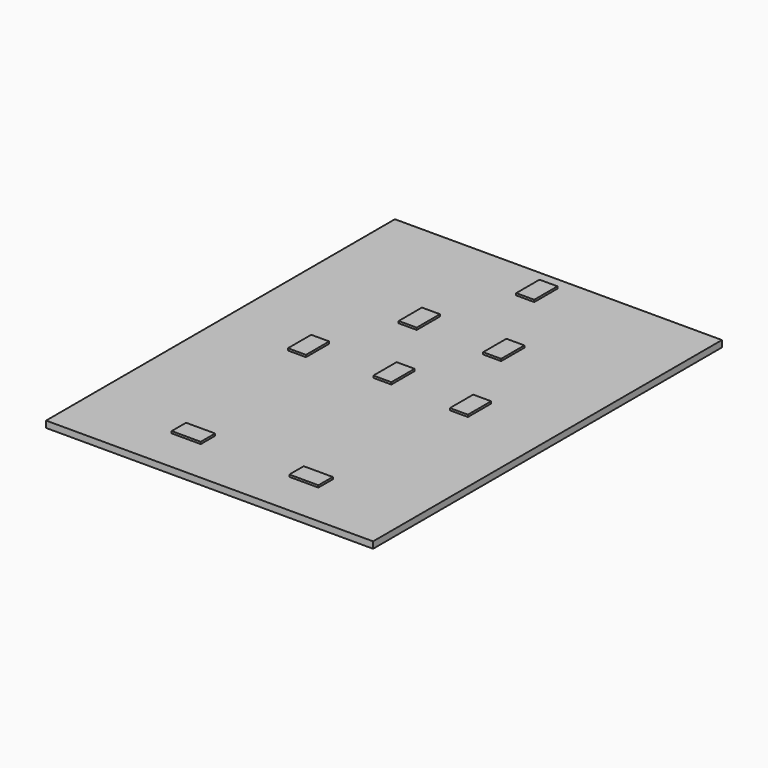
from build123d import *

# Parameters (mm, degrees)
F0_W     = 1500
F0_H     = 2000
F1_DEPTH = 5
F2_W     = 1480
F2_H     = 1980
F3_DEPTH = 20
F4_DEPTH = 20
F5_W     = 1500
F5_H     = 2000
F6_DEPTH = 5
F7_W     = 76.2
F7_H     = 130.175
F8_DEPTH = 9.525
F7_W_2   = 130.175
F7_H_2   = 76.2
F7_W_3   = 38.1


# Not quite as in the source:
# - a feature of the source that left no trace in its solid (it failed there, or was rolled back) is left out


with BuildPart() as f1:
    # F0 (on Top) → F1 (new body)
    with BuildSketch(Plane.XY):
        with Locations((750, 1000)):
            Rectangle(F0_W, F0_H)
    extrude(amount=F1_DEPTH)

    # F2 (on face) → F4 (join)
    with BuildSketch(Plane.XY.offset(5)):
        Polygon((0, 2000), (0, 0), (10, 0), (10, 10), (10, 1990), (1490, 1990), (1500, 1990), (1500, 2000), align=None)
        Polygon((10, 10), (10, 0), (1500, 0), (1500, 1990), (1490, 1990), (1490, 10), align=None)
    extrude(amount=F4_DEPTH)

    # F5 (on face) → F6 (join)
    with BuildSketch(Plane.XY.offset(25)):
        with Locations((750, 1000)):
            Rectangle(F5_W, F5_H)
    extrude(amount=F6_DEPTH)


with BuildPart() as f3:
    # F2 (on face) → F3 (new body)
    with BuildSketch(Plane.XY.offset(5)):
        with Locations((750, 1000)):
            Rectangle(F2_W, F2_H)
    extrude(amount=F3_DEPTH)


with BuildPart() as f8:
    # F7 (on face) → F8 (new body)
    with BuildSketch(Plane.XY.offset(30)):
        Polygon((594.425, 1377.95), (597.6, 1377.95), (597.6, 1511.3), (515.05, 1511.3), (515.05, 1377.95), (518.225, 1377.95), (518.225, 1508.125), (594.425, 1508.125), align=None)
        with Locations((556.325, 1443.0375)):
            Rectangle(F7_W, F7_H)
    extrude(amount=F8_DEPTH)


with BuildPart() as f8b:
    # F7 (on face) → F8, piece 2 (new body)
    with BuildSketch(Plane.XY.offset(30)):
        with Locations((943.675, 1443.0375)):
            Rectangle(F7_W, F7_H)
        Polygon((902.4, 1511.3), (902.4, 1377.95), (905.575, 1377.95), (905.575, 1508.125), (981.775, 1508.125), (981.775, 1377.95), (984.95, 1377.95), (984.95, 1511.3), align=None)
    extrude(amount=F8_DEPTH)


with BuildPart() as f8c:
    # F7 (on face) → F8, piece 3 (new body)
    with BuildSketch(Plane.XY.offset(30)):
        Polygon((708.725, 1809.75), (711.9, 1809.75), (711.9, 1939.925), (788.1, 1939.925), (788.1, 1809.75), (791.275, 1809.75), (791.275, 1943.1), (708.725, 1943.1), align=None)
        Polygon((711.9, 1809.75), (750, 1809.75), (788.1, 1809.75), (788.1, 1939.925), (711.9, 1939.925), align=None)
    extrude(amount=F8_DEPTH)


with BuildPart() as f8d:
    # F7 (on face) → F8, piece 4 (new body)
    with BuildSketch(Plane.XY.offset(30)):
        Polygon((419.8, 965.2), (419.8, 990.6), (419.8, 1098.55), (416.625, 1098.55), (416.625, 968.375), (340.425, 968.375), (340.425, 1098.55), (337.25, 1098.55), (337.25, 965.2), align=None)
        with Locations((378.525, 1033.4625)):
            Rectangle(F7_W, F7_H)
    extrude(amount=F8_DEPTH)


with BuildPart() as f8e:
    # F7 (on face) → F8, piece 5 (new body)
    with BuildSketch(Plane.XY.offset(30)):
        with Locations((481.7125, 244.475)):
            Rectangle(F7_W_2, F7_H_2)
        Polygon((413.45, 203.2), (546.8, 203.2), (546.8, 206.375), (416.625, 206.375), (416.625, 282.575), (546.8, 282.575), (546.8, 285.75), (413.45, 285.75), align=None)
    extrude(amount=F8_DEPTH)


with BuildPart() as f8f:
    # F7 (on face) → F8, piece 6 (new body)
    with BuildSketch(Plane.XY.offset(30)):
        with Locations((1018.2875, 244.475)):
            Rectangle(F7_W_2, F7_H_2)
        Polygon((953.2, 206.375), (953.2, 203.2), (1086.55, 203.2), (1086.55, 285.75), (953.2, 285.75), (953.2, 282.575), (1083.375, 282.575), (1083.375, 206.375), align=None)
    extrude(amount=F8_DEPTH)


with BuildPart() as f8g:
    # F7 (on face) → F8, piece 7 (new body)
    with BuildSketch(Plane.XY.offset(30)):
        Polygon((1080.2, 1098.55), (1080.2, 990.6), (1080.2, 965.2), (1162.75, 965.2), (1162.75, 1098.55), (1159.575, 1098.55), (1159.575, 968.375), (1083.375, 968.375), (1083.375, 1098.55), align=None)
        with Locations((1121.475, 1033.4625)):
            Rectangle(F7_W, F7_H)
    extrude(amount=F8_DEPTH)


with BuildPart() as f8h:
    # F7 (on face) → F8, piece 8 (new body)
    with BuildSketch(Plane.XY.offset(30)):
        with Locations((730.95, 1058.8625)):
            Rectangle(F7_W_3, F7_H)
        Polygon((708.725, 990.6), (750, 990.6), (750, 993.775), (711.9, 993.775), (711.9, 1123.95), (708.725, 1123.95), align=None)
        Polygon((750, 993.775), (750, 990.6), (791.275, 990.6), (791.275, 1123.95), (788.1, 1123.95), (788.1, 993.775), align=None)
        with Locations((769.05, 1058.8625)):
            Rectangle(F7_W_3, F7_H)
    extrude(amount=F8_DEPTH)


solid = Compound([f1.part, f3.part, f8.part, f8b.part, f8c.part, f8d.part, f8e.part, f8f.part, f8g.part, f8h.part])
